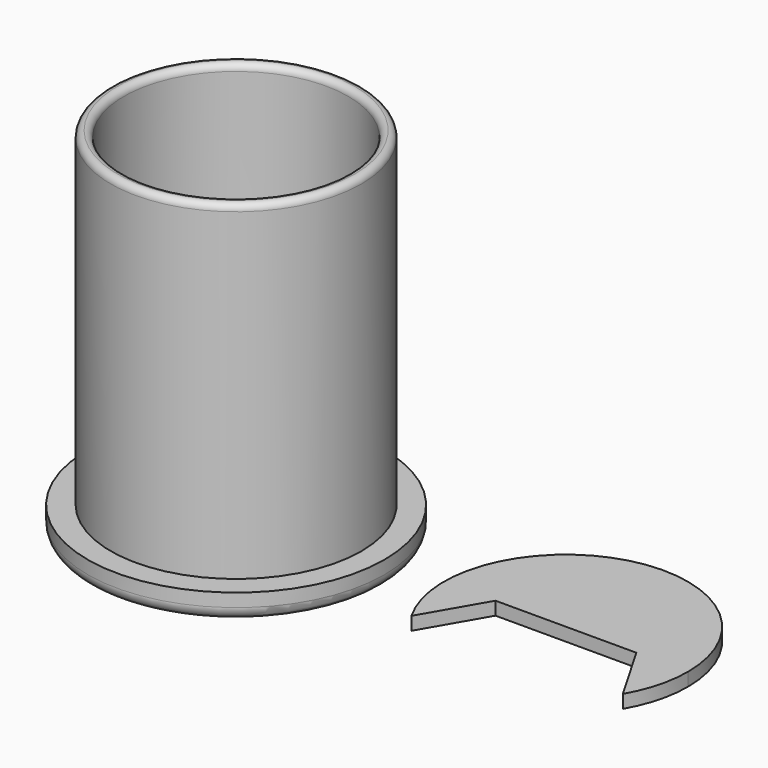
from build123d import *

# Parameters (mm, degrees)
F0_R          = 19
F0_R_2        = 17
F1_DEPTH      = 52
F0_R_3        = 22.5
F2_DEPTH      = 2
F2_DEPTH_BACK = 2
F3_R          = 1.99999
F4_R          = 0.99999
F5_DEPTH      = 2
F6_R          = 0.5


# Not quite as in the source:
# - a fillet or chamfer is up to 0.001 mm smaller than in the source, because OpenCascade refuses the exact size


with BuildPart() as f1:
    # F0 (on Top) → F1 (new body)
    with BuildSketch(Plane.XY):
        Circle(F0_R)
        Circle(F0_R_2, mode=Mode.SUBTRACT)
    extrude(amount=F1_DEPTH)

    # F0 (on Top) → F2 (join, two sides)
    with BuildSketch(Plane.XY) as f2_sk:
        Circle(F0_R_3)
        Circle(F0_R, mode=Mode.SUBTRACT)
    extrude(amount=F2_DEPTH)
    extrude(f2_sk.sketch, amount=-F2_DEPTH_BACK)

    # F3 (radius 2 in the source; OpenCascade refuses exactly that, so slightly less here)
    f3_edges = [f1.edges().sort_by_distance(p)[0] for p in [
        (-22.5, 0, -2),
    ]]
    fillet(f3_edges, radius=F3_R)

    # F4 (radius 1 in the source; OpenCascade refuses exactly that, so slightly less here)
    f4_edges = [f1.edges().sort_by_distance(p)[0] for p in [
        (-19, 0, 52),
        (-17, 0, 52),
    ]]
    fillet(f4_edges, radius=F4_R)

    # F6
    f6_edges = [f1.edges().sort_by_distance(p)[0] for p in [
        (-17, 0, 0),
    ]]
    fillet(f6_edges, radius=F6_R)


with BuildPart() as f5:
    # F0 (on Top) → F5 (new body)
    with BuildSketch(Plane.XY):
        with BuildLine():
            ThreePointArc((66.02146997, -9.25), (67.8696277863, -4.7881523344), (68.5, 0))
            ThreePointArc((68.5, 0), (45.2118476656, 17.8696277863), (33.97853003, -9.25))
            Line((33.97853003, -9.25), (39.31902002, 0))
            Line((39.31902002, 0), (60.68097998, 0))
            Line((60.68097998, 0), (66.02146997, -9.25))
        make_face()
    extrude(amount=F5_DEPTH)


solid = Compound([f1.part, f5.part])
